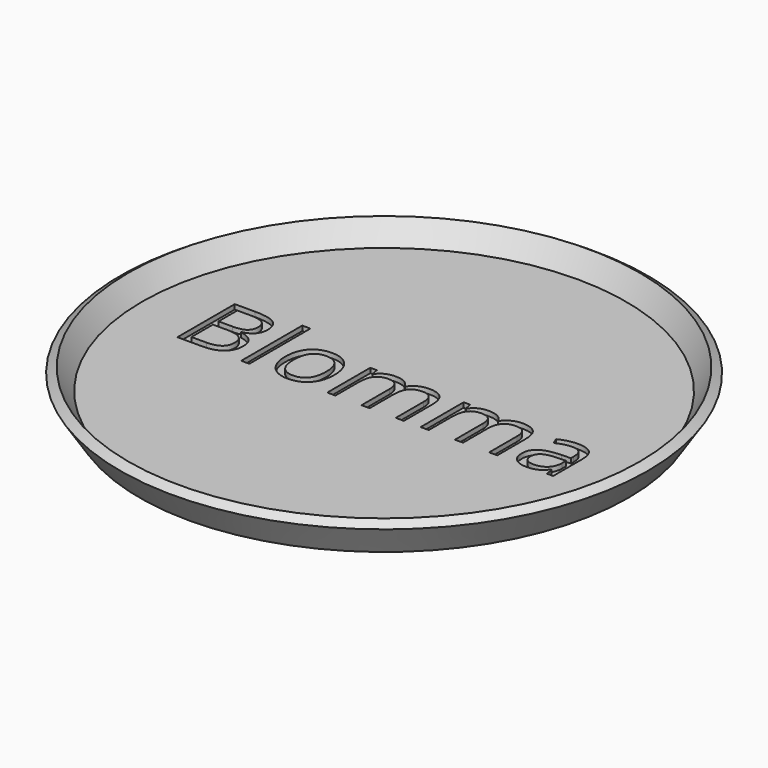
from build123d import *

# Parameters (mm, degrees)
F2_TEXT_SIZE = 20.8307905122
F3_DEPTH     = 1


# Not quite as in the source:
# - Text() gives the source's letters only with a copy of the font that has no kerning and outlines rounded to 1/6400 em; it was checked with that copy


with BuildPart() as f1:
    # F0 (on Front) → F1 (revolve)
    with BuildSketch(Plane.XZ):
        Polygon((0, 0), (50.7166795433, 0), (54.7659029411, 6.2441308979), (53.0446337681, 7.3603476337), (50.217015009, 3), (0, 3), align=None)
    revolve(axis=Axis((0, 0, 5.2361211143), (0, 0, 1)))

    # F2 (on face) → F3 (cut)
    with BuildSketch(Plane.XY.offset(3)):
        with Locations((-40, -6.1579736396)):
            Text('Blomma', F2_TEXT_SIZE, font='Open Sans', text_align=(TextAlign.LEFT, TextAlign.BOTTOM))
    extrude(amount=-F3_DEPTH, mode=Mode.SUBTRACT)


solid = f1.part
